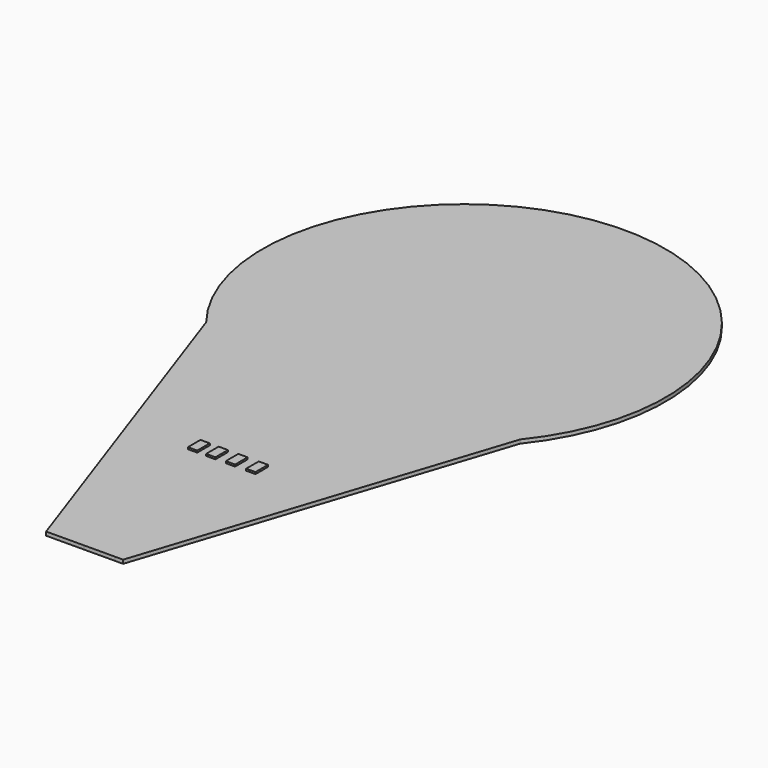
from build123d import *

# Parameters (mm, degrees)
F0_W     = 6.3504016859
F0_H     = 10.7357241213
F5_DEPTH = 3.81
F6_DEPTH = 2.54


# Not quite as in the source:
# - the program builds the solid bodies; features that only make, move or delete a surface that nothing else refers to are left out


with BuildPart() as f5:
    # F0 (on Top) → F5 (new body)
    with BuildSketch(Plane.XY):
        with Locations((20.3327481219, 62.6413132995)):
            Rectangle(F0_W, F0_H)
    extrude(amount=F5_DEPTH)


with BuildPart() as f5b:
    # F0 (on Top) → F5, piece 2 (new body)
    with BuildSketch(Plane.XY):
        with Locations((32.7791477969, 62.6413132995)):
            Rectangle(F0_W, F0_H)
    extrude(amount=F5_DEPTH)


with BuildPart() as f5c:
    # F0 (on Top) → F5, piece 3 (new body)
    with BuildSketch(Plane.XY):
        with Locations((46.2415534487, 62.6413132995)):
            Rectangle(F0_W, F0_H)
    extrude(amount=F5_DEPTH)


with BuildPart() as f5d:
    # F0 (on Top) → F5, piece 4 (new body)
    with BuildSketch(Plane.XY):
        with Locations((60.2119545868, 62.6413132995)):
            Rectangle(F0_W, F0_H)
    extrude(amount=F5_DEPTH)


with BuildPart() as f6:
    # F0 (on Top) → F6 (new body)
    with BuildSketch(Plane.XY):
        with BuildLine():
            Line((69.9580198012, -64.1605830248), (148.7393677235, 177.0247817039))
            ThreePointArc((148.7393677235, 177.0247817039), (41.9997875967, 401.1840791368), (-67.0538321137, 178.141400218))
            Line((-67.0538321137, 178.141400218), (17.4566285457, -64.4657063324))
            Line((17.4566285457, -64.4657063324), (23.8170791066, -64.4287411841))
            Line((23.8170791066, -64.4287411841), (43.1908853352, -64.3161460757))
            Line((43.1908853352, -64.3161460757), (64.2538569655, -64.1937340135))
            Line((64.2538569655, -64.1937340135), (69.9580198012, -64.1605830248))
        make_face()
        with Locations((20.3327481219, 62.6413132995)):
            Rectangle(F0_W, F0_H, mode=Mode.SUBTRACT)
        with Locations((32.7791477969, 62.6413132995)):
            Rectangle(F0_W, F0_H, mode=Mode.SUBTRACT)
        with Locations((46.2415534487, 62.6413132995)):
            Rectangle(F0_W, F0_H, mode=Mode.SUBTRACT)
        with Locations((60.2119545868, 62.6413132995)):
            Rectangle(F0_W, F0_H, mode=Mode.SUBTRACT)
    extrude(amount=F6_DEPTH)


solid = Compound([f5.part, f5b.part, f5c.part, f5d.part, f6.part])
